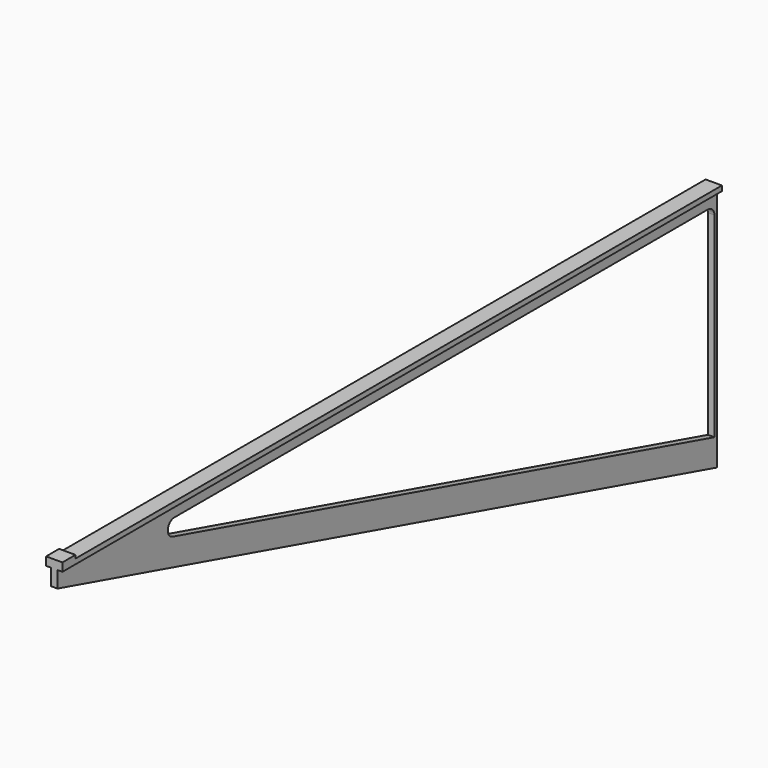
from build123d import *

# Parameters (mm, degrees)
F1_DEPTH = 505
F2_W     = 10
F2_H     = 10
F3_DEPTH = 2
F5_DEPTH = 25
F7_DEPTH = 25
F8_R     = 5


with BuildPart() as f1:
    # F0 (on Front) → F1 (new body)
    with BuildSketch(Plane.XZ):
        Polygon((3, 5.9644671453), (-7, 5.9644671453), (-7, 2.8680202551), (-4, 2.8680202551), (-4, -147.1319797449), (0, -147.1319797449), (0, 2.8680202551), (3, 2.8680202551), align=None)
    extrude(amount=F1_DEPTH)

    # F2 (on face) → F3 (join)
    with BuildSketch(Plane.XY.offset(5.9644671453)):
        with Locations((-2, -500)):
            Rectangle(F2_W, F2_H)
    extrude(amount=F3_DEPTH)

    # F4 (on face) → F5 (cut)
    with BuildSketch(Plane(origin=(-4, 0, 0), x_dir=(0, -1, 0), z_dir=(-1, 0, 0))):
        Polygon((505, -147.1319797449), (505, -7.1319797449), (0, -147.1319797449), align=None)
    extrude(amount=-F5_DEPTH, mode=Mode.SUBTRACT)

    # F6 (on face) → F7 (cut)
    with BuildSketch(Plane(origin=(-4, 0, 0), x_dir=(0, -1, 0), z_dir=(-1, 0, 0))):
        Polygon((452.3232281555, -5.1319797449), (2, -5.1319797449), (2, -129.9740627979), align=None)
    extrude(amount=-F7_DEPTH, mode=Mode.SUBTRACT)

    # F8
    f8_edges = [f1.edges().sort_by_distance(p)[0] for p in [
        (-2, -2, -5.13198),
        (-2, -452.323228, -5.13198),
    ]]
    fillet(f8_edges, radius=F8_R)


solid = f1.part
